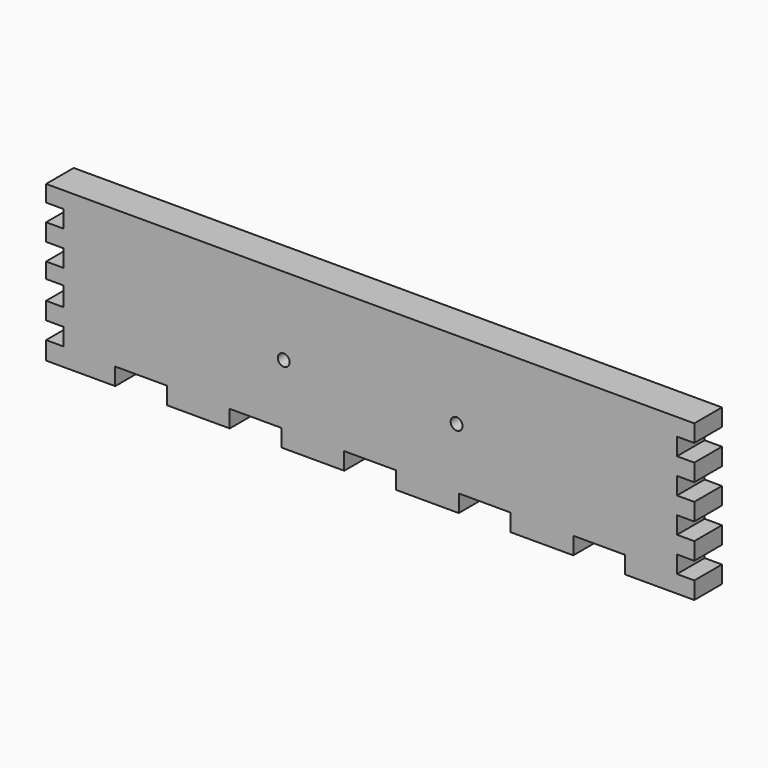
from build123d import *

# Parameters (mm, degrees)
F0_R     = 4.7625
F1_DEPTH = 12.7
F2_START = 1.5875
F0_R_2   = 2.1844
F2_DEPTH = 11.1125
F3_START = 1.5875
F3_DEPTH = 11.1125


# Not quite as in the source:
# - a feature names something its author has since deleted; it is built from what else it names


with BuildPart() as f1:
    # F0 (on Front) → F1 (new body)
    with BuildSketch(Plane.XZ):
        Polygon((97.3731166124, 28.1938837487), (97.3731166124, 34.5438837487), (-140.7518833876, 34.5438837487), (-140.7518833876, 28.5026916087), (-134.4018833876, 28.5026916087), (-134.4018833876, 22.1526916087), (-140.7518833876, 22.1526916087), (-140.7518833876, 15.8026916087), (-134.4018833876, 15.8026916087), (-134.4018833876, 9.4526916087), (-140.7518833876, 9.4526916087), (-140.7518833876, 3.7844837487), (-134.4018833876, 3.7844837487), (-134.4018833876, -3.2473083913), (-140.7518833876, -3.2473083913), (-140.7518833876, -9.5973083913), (-134.4018833876, -9.5973083913), (-134.4018833876, -15.9473083913), (-140.7518833876, -15.9473083913), (-140.7518833876, -22.6061162513), (-115.3518833876, -22.6061162513), (-115.3518833876, -16.2561162513), (-96.3018833876, -16.2561162513), (-96.3018833876, -22.6061162513), (-73.2831333876, -22.6061162513), (-73.2831333876, -16.2561162513), (-54.2331333876, -16.2561162513), (-54.2331333876, -22.6061162513), (-31.2143833876, -22.6061162513), (-31.2143833876, -16.2561162513), (-12.1643833876, -16.2561162513), (-12.1643833876, -22.6061162513), (10.8543666124, -22.6061162513), (10.8543666124, -16.2561162513), (29.9043666124, -16.2561162513), (29.9043666124, -22.6061162513), (52.9231166124, -22.6061162513), (52.9231166124, -16.2561162513), (71.9731166124, -16.2561162513), (71.9731166124, -22.6061162513), (97.3731166124, -22.6061162513), (97.3731166124, -16.2561162513), (91.0231166124, -16.2561162513), (91.0231166124, -9.9061162513), (97.3731166124, -9.9061162513), (97.3731166124, -3.5561162513), (91.0231166124, -3.5561162513), (91.0231166124, 2.7938837487), (97.3731166124, 2.7938837487), (97.3731166124, 9.1438837487), (91.0231166124, 9.1438837487), (91.0231166124, 15.4938837487), (97.3731166124, 15.4938837487), (97.3731166124, 21.8438837487), (91.0231166124, 21.8438837487), (91.0231166124, 28.1938837487), align=None)
        with Locations((-53.4393833876, 5.9688837487)):
            Circle(F0_R, mode=Mode.SUBTRACT)
        with Locations((10.0606166124, 5.9688837487)):
            Circle(F0_R, mode=Mode.SUBTRACT)
    extrude(amount=F1_DEPTH)

    # F0 (on Front) → F2 (join)
    with BuildSketch(Plane.XZ.offset(F2_START)):
        with Locations((-53.4393833876, 5.9688837487)):
            Circle(F0_R)
        with Locations((-53.4393833876, 5.9688837487)):
            Circle(F0_R_2, mode=Mode.SUBTRACT)
    extrude(amount=F2_DEPTH)

    # F0 (on Front) → F3 (join)
    with BuildSketch(Plane.XZ.offset(F3_START)):
        with Locations((10.0606166124, 5.9688837487)):
            Circle(F0_R)
        with Locations((10.0606166124, 5.9688837487)):
            Circle(F0_R_2, mode=Mode.SUBTRACT)
    extrude(amount=F3_DEPTH)


solid = f1.part
